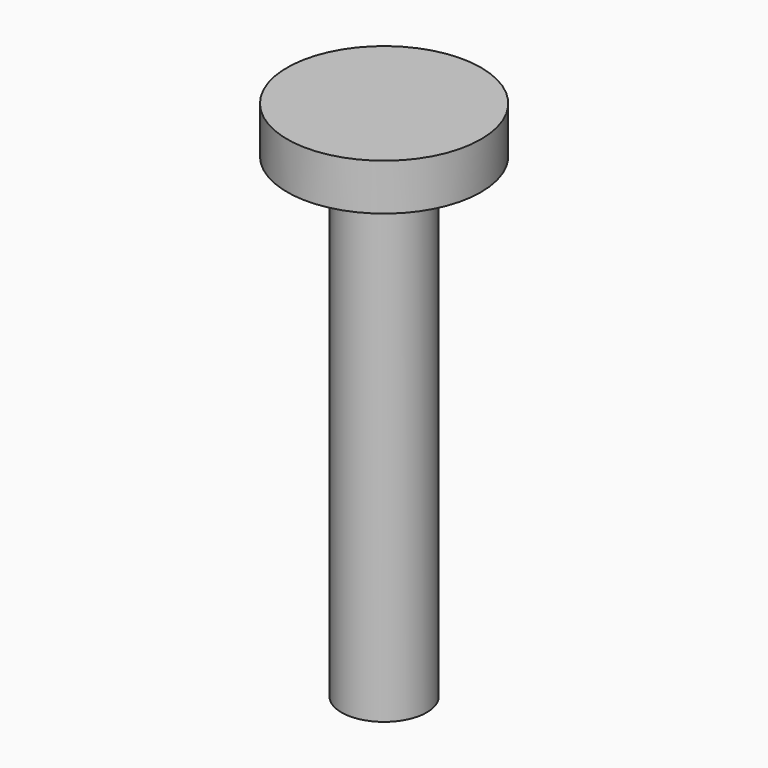
from build123d import *

# Parameters (mm, degrees)
F0_R          = 2.75
F1_DEPTH      = 32.1564
F2_R          = 6.25
F2_R_2        = 2.75
F3_DEPTH      = 1.5
F3_DEPTH_BACK = 1.5


with BuildPart() as f1:
    # F0 (on Top) → F1 (new body)
    with BuildSketch(Plane.XY):
        Circle(F0_R)
    extrude(amount=F1_DEPTH)

    # F2 (on face) → F3 (join, two sides)
    with BuildSketch(Plane.XY.offset(32.1564)) as f3_sk:
        Circle(F2_R)
        Circle(F2_R_2, mode=Mode.SUBTRACT)
        Circle(F2_R_2)
    extrude(amount=F3_DEPTH)
    extrude(f3_sk.sketch, amount=-F3_DEPTH_BACK)


solid = f1.part
